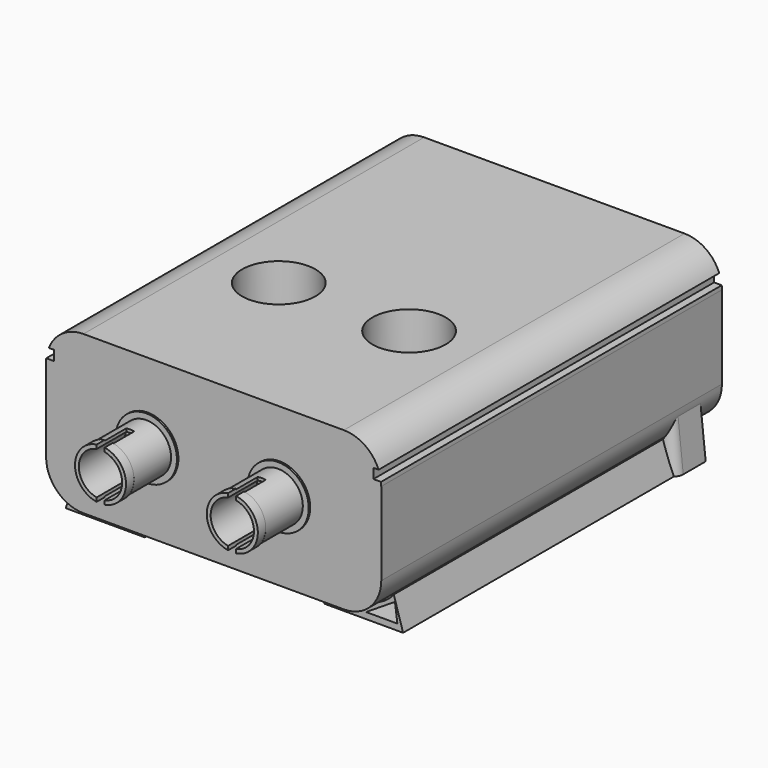
from build123d import *

# Parameters (mm, degrees)
F0_W            = 45.5422
F0_H            = 57.8612
F1_DEPTH        = 21.4376
F2_R            = 5.08
F3_R            = 4.1656
F4_DEPTH        = 0.254
F5_R            = 3.3655
F6_DEPTH        = 6.4262
F7_R            = 3.4671
F8_DEPTH        = 1.3462
F9_W            = 1.0922
F9_H            = 7.4237788019
F10_DEPTH       = 21.4386
F11_R           = 2.9415835505
F12_DEPTH       = 7.7724
F14_D           = 6.731
F14_DEPTH       = 8.0772
F14_CSINK_D     = 8.4836
F14_CSINK_ANGLE = 82
F14_TIP         = 2.0221964133
F15_R           = 4.9784
F16_DEPTH       = 8.0264
F18_DEPTH       = 25.4
F18_DEPTH_BACK  = 25.4
F20_DEPTH       = 62.358
F22_DEPTH       = 45.72
F23_R           = 1.27
F24_R           = 1.27
F26_R           = 3.5084573534
F26_R_2         = 3.3655
F27_DEPTH       = 1.27
F27_DEPTH_BACK  = 1.27
F29_DEPTH       = 65.8886


# Not quite as in the source:
# - a feature names something its author has since deleted; it is built from what else it names


with BuildPart() as f1:
    # F0 (on Top) → F1 (new body)
    with BuildSketch(Plane.XY):
        Rectangle(F0_W, F0_H)
    extrude(amount=F1_DEPTH)

    # F2
    f2_edges = [f1.edges().sort_by_distance(p)[0] for p in [
        (-22.7711, 0, 21.4376),
        (22.7711, 0, 21.4376),
        (22.7711, 0, 0),
        (-22.7711, 0, 0),
    ]]
    fillet(f2_edges, radius=F2_R)

    # F3 (on face) → F4 (join)
    with BuildSketch(Plane.XZ.offset(28.9306)):
        with Locations((-8.9535, 10.7188)):
            Circle(F3_R)
        with Locations((8.9535, 10.7188)):
            Circle(F3_R)
    extrude(amount=F4_DEPTH)

    # F5 (on face) → F6 (join)
    with BuildSketch(Plane.XZ.offset(29.1846)):
        with Locations((-8.9535, 10.7188)):
            Circle(F5_R)
        with Locations((8.9535, 10.7188)):
            Circle(F5_R)
    extrude(amount=F6_DEPTH)

    # F7 (on face) → F8 (join)
    with BuildSketch(Plane.XZ.offset(35.6108)):
        with Locations((-8.9535, 10.7188)):
            Circle(F7_R)
        with Locations((8.9535, 10.7188)):
            Circle(F7_R)
    extrude(amount=F8_DEPTH)

    # F9 (on Top) → F10 (cut, through all)
    with BuildSketch(Plane.XY):
        with Locations((-8.9281, -35.6396894009)):
            Rectangle(F9_W, F9_H)
        with Locations((8.9281, -35.6396894009)):
            Rectangle(F9_W, F9_H)
    extrude(amount=F10_DEPTH, mode=Mode.SUBTRACT)

    # F11 (on face) → F12 (cut, through all)
    with BuildSketch(Plane.XZ.offset(36.957)):
        with Locations((-8.9535, 10.7188)):
            Circle(F11_R)
        with Locations((8.9535, 10.7188)):
            Circle(F11_R)
    extrude(amount=-F12_DEPTH, mode=Mode.SUBTRACT)

    # F14
    with Locations(Plane(origin=(0, 28.9306, 0), x_dir=(-1, 0, 0), z_dir=(0, 1, 0))):
        with Locations((-9.0043, 10.7188), (9.0043, 10.7188)):
            CounterSinkHole(F14_D / 2, F14_CSINK_D / 2, depth=F14_DEPTH, counter_sink_angle=F14_CSINK_ANGLE)
            with Locations((0, 0, -(F14_DEPTH + F14_TIP / 2))):  # 118° drill point
                Cone(0, F14_D / 2, F14_TIP, mode=Mode.SUBTRACT)

    # F15 (on face) → F16 (cut)
    with BuildSketch(Plane.XY.offset(21.4376)):
        with Locations((-8.8519, -6.8072)):
            Circle(F15_R)
        with Locations((8.8519, -6.8072)):
            Circle(F15_R)
    extrude(amount=-F16_DEPTH, mode=Mode.SUBTRACT)

    # F26 (on offset) → F27 (cut, two sides)
    with BuildSketch(Plane(origin=(0, 20.9042, 0), x_dir=(-1, 0, 0), z_dir=(0, 1, 0))) as f27_sk:
        with Locations((-9.0043, 10.7188)):
            Circle(F26_R)
        with Locations((-9.0043, 10.7188)):
            Circle(F26_R_2, mode=Mode.SUBTRACT)
        with Locations((9.0043, 10.7188)):
            Circle(F26_R)
        with Locations((9.0043, 10.7188)):
            Circle(F26_R_2, mode=Mode.SUBTRACT)
    extrude(amount=-F27_DEPTH, mode=Mode.SUBTRACT)
    extrude(f27_sk.sketch, amount=F27_DEPTH_BACK, mode=Mode.SUBTRACT)

    # F28 (on face) → F29 (cut, through all)
    with BuildSketch(Plane(origin=(0, 28.9306, 0), x_dir=(-1, 0, 0), z_dir=(0, 1, 0))):
        with BuildLine():
            ThreePointArc((-22.7430188869, 16.891), (-22.622948443, 17.5754961103), (-22.4105813105, 18.2372))
            Line((-22.4105813105, 18.2372), (-22.7711, 18.2372))
            Line((-22.7711, 18.2372), (-22.7711, 16.891))
            Line((-22.7711, 16.891), (-22.7430188869, 16.891))
        make_face()
        with BuildLine():
            Line((22.7711, 16.891), (22.7711, 18.2372))
            Line((22.7711, 18.2372), (22.4105813105, 18.2372))
            ThreePointArc((22.4105813105, 18.2372), (22.622948443, 17.5754961103), (22.7430188869, 16.891))
            Line((22.7430188869, 16.891), (22.7711, 16.891))
        make_face()
        with BuildLine():
            ThreePointArc((22.7430188869, 16.891), (22.622948443, 17.5754961103), (22.4105813105, 18.2372))
            Line((22.4105813105, 18.2372), (21.7043, 18.2372))
            Line((21.7043, 18.2372), (21.7043, 16.891))
            Line((21.7043, 16.891), (22.7430188869, 16.891))
        make_face()
        with BuildLine():
            Line((-21.7043, 18.2372), (-22.4105813105, 18.2372))
            ThreePointArc((-22.4105813105, 18.2372), (-22.622948443, 17.5754961103), (-22.7430188869, 16.891))
            Line((-22.7430188869, 16.891), (-21.7043, 16.891))
            Line((-21.7043, 16.891), (-21.7043, 18.2372))
        make_face()
    extrude(amount=-F29_DEPTH, mode=Mode.SUBTRACT)


with BuildPart() as f18:
    # F17 (on Front) → F18 (new body, two sides)
    with BuildSketch(Plane.XZ) as f18_sk:
        with BuildLine():
            Line((-22.6860410745, 4.1542766816), (-23.3881954099, -2.54))
            Line((-23.3881954099, -2.54), (-12.1926218763, -2.54))
            Line((-12.1926218763, -2.54), (-13.9572033659, 0))
            Line((-13.9572033659, 0), (-19.4434244186, 0))
            ThreePointArc((-19.4434244186, 0), (-21.64555842, 1.6237754217), (-22.6860410745, 4.1542766816))
        make_face()
    extrude(amount=F18_DEPTH)
    extrude(f18_sk.sketch, amount=-F18_DEPTH_BACK)


with BuildPart() as f18b:
    # F17 (on Front) → F18, piece 2 (new body, two sides)
    with BuildSketch(Plane.XZ) as f18_2_sk:
        with BuildLine():
            Line((23.3881954099, -2.54), (22.6860410745, 4.1542766816))
            ThreePointArc((22.6860410745, 4.1542766816), (21.64555842, 1.6237754217), (19.4434244186, 0))
            Line((19.4434244186, 0), (13.9572033659, 0))
            Line((13.9572033659, 0), (12.1926218763, -2.54))
            Line((12.1926218763, -2.54), (23.3881954099, -2.54))
        make_face()
    extrude(amount=F18_DEPTH)
    extrude(f18_2_sk.sketch, amount=-F18_DEPTH_BACK)


with BuildPart() as f20_tool:
    # F19 (on face) → F20 (new body, through all)
    with BuildSketch(Plane(origin=(0, 25.4, 0), x_dir=(-1, 0, 0), z_dir=(0, 1, 0))):
        Polygon((-17.8844314561, -1.6902784118), (-21.8110085026, 0.8071383408), (-22.1399367348, -1.6902784118), align=None)
        Polygon((17.8844314561, -1.6902784118), (22.1399367348, -1.6902784118), (21.8110085026, 0.8071383408), align=None)
    extrude(amount=-F20_DEPTH)


with BuildPart() as f18_1:
    add(f18.part)

    # F20: cut by f20_tool
    add(f20_tool.part, mode=Mode.SUBTRACT)


with BuildPart() as f18b_1:
    add(f18b.part)

    # F20: cut by f20_tool
    add(f20_tool.part, mode=Mode.SUBTRACT)


with BuildPart() as f22_tool:
    # F21 (on face) → F22 (new body)
    with BuildSketch(Plane.XZ.offset(25.4)):
        with BuildLine():
            ThreePointArc((-21.64555842, 1.6237754217), (-22.3393702945, 2.8176579213), (-22.6860410745, 4.1542766816))
            Line((-22.6860410745, 4.1542766816), (-24.1758879766, -3.2762847841))
            Line((-24.1758879766, -3.2762847841), (-23.0863132075, -3.0912626535))
            Line((-23.0863132075, -3.0912626535), (-21.64555842, 1.6237754217))
        make_face()
        with BuildLine():
            Line((21.64555842, 1.6237754217), (23.0863132075, -3.0912626535))
            Line((23.0863132075, -3.0912626535), (24.1758879766, -3.2762847841))
            Line((24.1758879766, -3.2762847841), (22.6860410745, 4.1542766816))
            ThreePointArc((22.6860410745, 4.1542766816), (22.3393702945, 2.8176579213), (21.64555842, 1.6237754217))
        make_face()
    extrude(amount=-F22_DEPTH)


with BuildPart() as f18_2:
    add(f18_1.part)

    # F22: cut by f22_tool
    add(f22_tool.part, mode=Mode.SUBTRACT)

    # F23
    f23_edges = [f18_2.edges().sort_by_distance(p)[0] for p in [
        (-23.037118, 20.32, 0.807138),
    ]]
    fillet(f23_edges, radius=F23_R)


with BuildPart() as f18b_2:
    add(f18b_1.part)

    # F22: cut by f22_tool
    add(f22_tool.part, mode=Mode.SUBTRACT)

    # F24
    f24_edges = [f18b_2.edges().sort_by_distance(p)[0] for p in [
        (23.037118, 20.32, 0.807138),
    ]]
    fillet(f24_edges, radius=F24_R)


solid = Compound([f1.part, f18_2.part, f18b_2.part])
